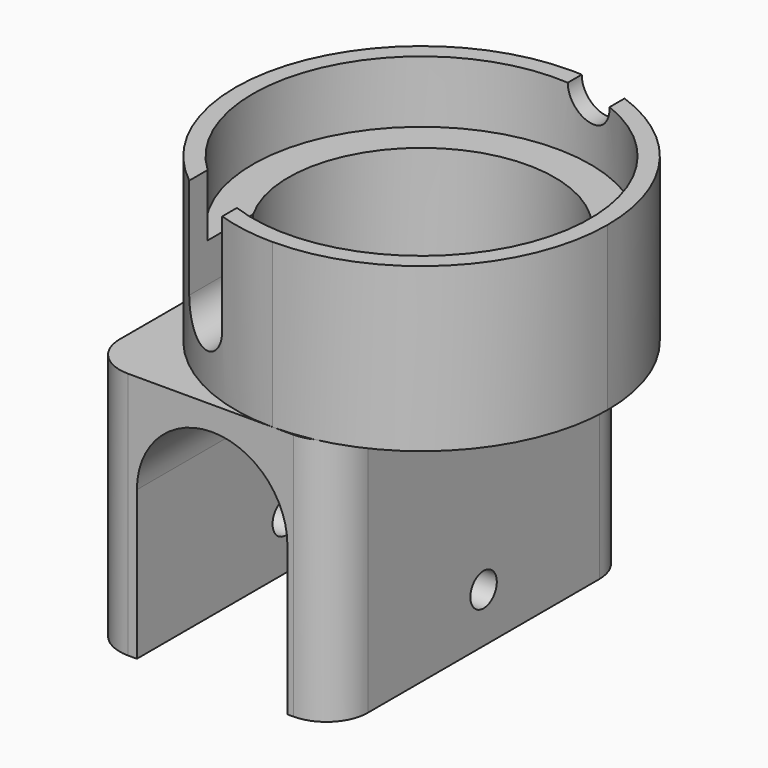
from build123d import *

# Parameters (mm, degrees)
F0_W      = 45
F0_H      = 45
F1_DEPTH  = 19.7
F2_R      = 20.4
F3_DEPTH  = 7.5
F4_R      = 16.1
F5_DEPTH  = 12.2
F7_DEPTH  = 14.5505284159
F9_DEPTH  = 3.5695447941
F11_DEPTH = 30
F13_DEPTH = 45
F14_R     = 22.49999
F16_DEPTH = 2
F17_R     = 2
F18_DEPTH = 43.0010001
F19_R     = 5
F20_R     = 1.5
F21_DEPTH = 7.5
F22_R     = 1.5
F23_DEPTH = 3


# Not quite as in the source:
# - a fillet or chamfer is up to 0.001 mm smaller than in the source, because OpenCascade refuses the exact size


with BuildPart() as f1:
    # F0 (on Top) → F1 (new body)
    with BuildSketch(Plane.XY):
        Rectangle(F0_W, F0_H)
    extrude(amount=F1_DEPTH)

    # F2 (on face) → F3 (cut)
    with BuildSketch(Plane.XY.offset(19.7)):
        Circle(F2_R)
    extrude(amount=-F3_DEPTH, mode=Mode.SUBTRACT)

    # F4 (on face) → F5 (cut, through all)
    with BuildSketch(Plane.XY.offset(12.2)):
        Circle(F4_R)
    extrude(amount=-F5_DEPTH, mode=Mode.SUBTRACT)

    # F6 (on face) → F7 (cut, through all)
    with BuildSketch(Plane.XZ.offset(22.5)):
        with BuildLine():
            Line((-14, 19.7), (-14, 7.5))
            ThreePointArc((-14, 7.5), (-10.5, 4), (-7, 7.5))
            Line((-7, 7.5), (-7, 19.7))
            Line((-7, 19.7), (-14, 19.7))
        make_face()
    extrude(amount=-F7_DEPTH, mode=Mode.SUBTRACT)

    # F8 (on face) → F9 (cut, through all)
    with BuildSketch(Plane(origin=(0, 22.5, 0), x_dir=(-1, 0, 0), z_dir=(0, 1, 0))):
        with BuildLine():
            Line((-1.4, 19.7), (-7.6, 19.7))
            ThreePointArc((-7.6, 19.7), (-4.5, 16.6), (-1.4, 19.7))
        make_face()
    extrude(amount=-F9_DEPTH, mode=Mode.SUBTRACT)

    # F14 (radius 22.5 in the source; OpenCascade refuses exactly that, so slightly less here)
    f14_edges = [f1.edges().sort_by_distance(p)[0] for p in [
        (22.5, -22.5, 9.85),
        (-22.5, -22.5, 9.85),
        (-22.5, 22.5, 9.85),
        (22.5, 22.5, 9.85),
    ]]
    fillet(f14_edges, radius=F14_R)


with BuildPart() as f11:
    # F10 (on face) → F11 (new body)
    with BuildSketch(Plane(origin=(0, 0, 0), x_dir=(1, 0, 0), z_dir=(0, 0, -1))):
        with BuildLine():
            Line((7.5, 22.5), (-22.5, 22.5))
            Line((-22.5, 22.5), (-22.5, -22.5))
            Line((-22.5, -22.5), (7.5, -22.5))
            Line((7.5, -22.5), (7.5, -14.2464030548))
            ThreePointArc((7.5, -14.2464030548), (-16.1, 0), (7.5, 14.2464030548))
            Line((7.5, 14.2464030548), (7.5, 22.5))
        make_face()
        with BuildLine():
            Line((7.5, -14.2464030548), (7.5, 14.2464030548))
            ThreePointArc((7.5, 14.2464030548), (-16.1, 0), (7.5, -14.2464030548))
        make_face()
    extrude(amount=F11_DEPTH)

    # F12 (on face) → F13 (cut, through all)
    with BuildSketch(Plane.XZ.offset(22.5)):
        with BuildLine():
            Line((1.7810865191, -30), (1.7810865191, -12))
            ThreePointArc((1.7810865191, -12), (-7.3189134809, -2.9), (-16.4189134809, -12))
            Line((-16.4189134809, -12), (-16.4189134809, -30))
            Line((-16.4189134809, -30), (1.7810865191, -30))
        make_face()
    extrude(amount=-F13_DEPTH, mode=Mode.SUBTRACT)

    # F15 (on face) → F16 (cut)
    with BuildSketch(Plane(origin=(-22.5, 0, 0), x_dir=(0, -1, 0), z_dir=(-1, 0, 0))):
        Polygon((-2, -27.4641016151), (2, -27.4641016151), (4, -24), (2, -20.5358983849), (-2, -20.5358983849), (-4, -24), align=None)
    extrude(amount=-F16_DEPTH, mode=Mode.SUBTRACT)

    # F17 (on face) → F18 (cut, through all)
    with BuildSketch(Plane(origin=(-20.5, 0, 0), x_dir=(0, -1, 0), z_dir=(-1, 0, 0))):
        with Locations((0, -24)):
            Circle(F17_R)
    extrude(amount=-F18_DEPTH, mode=Mode.SUBTRACT)

    # F19
    f19_edges = [f11.edges().sort_by_distance(p)[0] for p in [
        (-22.5, -22.5, -15),
        (7.5, -22.5, -15),
        (7.5, 22.5, -15),
        (-22.5, 22.5, -15),
    ]]
    fillet(f19_edges, radius=F19_R)

    # F20 (on face) → F21 (cut)
    with BuildSketch(Plane.XY):
        Circle(F20_R)
    extrude(amount=-F21_DEPTH, mode=Mode.SUBTRACT)

    # F22 (on face) → F23 (cut)
    with BuildSketch(Plane.XY):
        with Locations((-12, 0)):
            Circle(F22_R)
    extrude(amount=-F23_DEPTH, mode=Mode.SUBTRACT)


solid = Compound([f1.part, f11.part])
